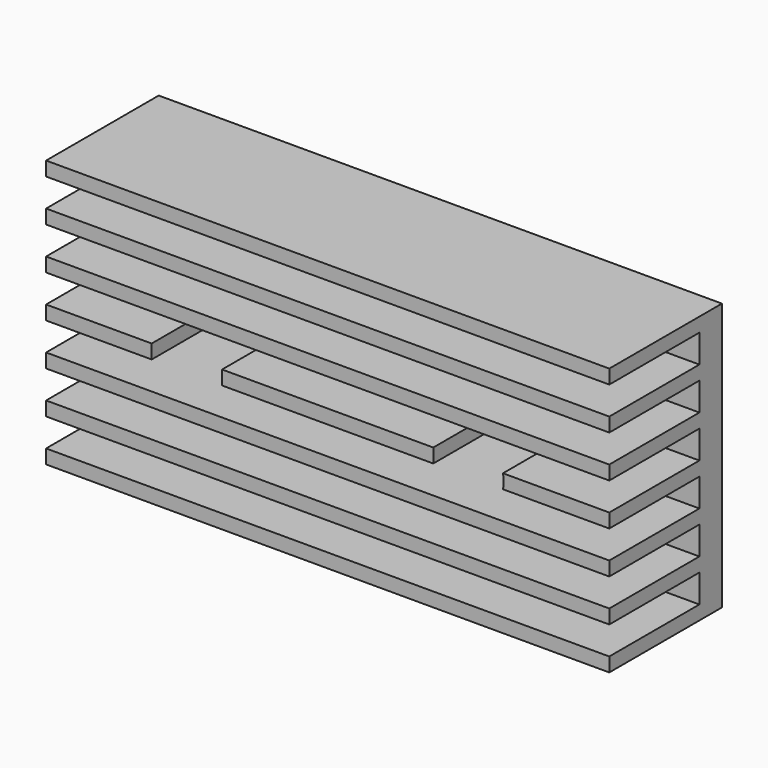
from build123d import *

# Parameters (mm, degrees)
F0_W     = 40
F0_H     = 19
F1_DEPTH = 10
F2_W     = 40
F2_H     = 2
F4_DEPTH = 8
F5_R     = 0.9
F5_W     = 4.6
F5_H     = 6.1
F7_DEPTH = 5
F8_DEPTH = 8.001
F9_DEPTH = 5.001


# Not quite as in the source:
# - a feature names something its author has since deleted; it is built from what else it names


with BuildPart() as f1:
    # F0 (on Front) → F1 (new body)
    with BuildSketch(Plane.XZ):
        Rectangle(F0_W, F0_H)
    extrude(amount=F1_DEPTH)

    # F2 (on face) → F4 (cut, through all)
    with BuildSketch(Plane.XZ.offset(10)):
        with Locations((0, 7.5)):
            Rectangle(F2_W, F2_H)
        with Locations((0, 4.5)):
            Rectangle(F2_W, F2_H)
        with Locations((0, 1.5)):
            Rectangle(F2_W, F2_H)
        with Locations((0, -1.5)):
            Rectangle(F2_W, F2_H)
        with Locations((0, -4.5)):
            Rectangle(F2_W, F2_H)
        with Locations((0, -7.5)):
            Rectangle(F2_W, F2_H)
    extrude(amount=-F4_DEPTH, mode=Mode.SUBTRACT)

    # F5 (on offset) → F7 (join, through all)
    with BuildSketch(Plane.XZ.offset(2)):
        with BuildLine():
            ThreePointArc((10, 2.5), (8.232233047, 1.767766953), (7.5, 0))
            ThreePointArc((7.5, 0), (8.232233047, -1.767766953), (10, -2.5))
            ThreePointArc((10, -2.5), (11.767766953, -1.767766953), (12.5, 0))
            ThreePointArc((12.5, 0), (11.767766953, 1.767766953), (10, 2.5))
        make_face()
        with Locations((10, 0)):
            Circle(F5_R, mode=Mode.SUBTRACT)
        with BuildLine():
            ThreePointArc((-10, -2.5), (-8.232233047, -1.767766953), (-7.5, 0))
            ThreePointArc((-7.5, 0), (-8.232233047, 1.767766953), (-10, 2.5))
            ThreePointArc((-10, 2.5), (-11.767766953, 1.767766953), (-12.5, 0))
            ThreePointArc((-12.5, 0), (-11.767766953, -1.767766953), (-10, -2.5))
        make_face()
        with Locations((-10, 0)):
            Circle(F5_R, mode=Mode.SUBTRACT)
        with Locations((0, -1.25)):
            Rectangle(F5_W, F5_H)
    extrude(amount=-F7_DEPTH)

    # F5 (on offset) → F8 (cut, through all)
    with BuildSketch(Plane.XZ.offset(2)):
        with BuildLine():
            ThreePointArc((-10, 2.5), (-8.232233047, 1.767766953), (-7.5, 0))
            Line((-7.5, 0), (-7.5, 2.5))
            Line((-7.5, 2.5), (-10, 2.5))
        make_face()
        with BuildLine():
            ThreePointArc((-12.5, 0), (-11.767766953, 1.767766953), (-10, 2.5))
            Line((-10, 2.5), (-12.5, 2.5))
            Line((-12.5, 2.5), (-12.5, 0))
        make_face()
        with BuildLine():
            Line((-12.5, -2.5), (-10, -2.5))
            ThreePointArc((-10, -2.5), (-11.767766953, -1.767766953), (-12.5, 0))
            Line((-12.5, 0), (-12.5, -2.5))
        make_face()
        with BuildLine():
            Line((-7.5, -2.5), (-7.5, 0))
            ThreePointArc((-7.5, 0), (-8.232233047, -1.767766953), (-10, -2.5))
            Line((-10, -2.5), (-7.5, -2.5))
        make_face()
        with BuildLine():
            ThreePointArc((-10, -2.5), (-8.232233047, -1.767766953), (-7.5, 0))
            ThreePointArc((-7.5, 0), (-8.232233047, 1.767766953), (-10, 2.5))
            ThreePointArc((-10, 2.5), (-11.767766953, 1.767766953), (-12.5, 0))
            ThreePointArc((-12.5, 0), (-11.767766953, -1.767766953), (-10, -2.5))
        make_face()
        with Locations((-10, 0)):
            Circle(F5_R, mode=Mode.SUBTRACT)
        with Locations((-10, 0)):
            Circle(F5_R)
        with BuildLine():
            Line((10, 2.5), (7.5, 2.5))
            Line((7.5, 2.5), (7.5, 0))
            ThreePointArc((7.5, 0), (8.232233047, 1.767766953), (10, 2.5))
        make_face()
        with BuildLine():
            ThreePointArc((10, -2.5), (8.232233047, -1.767766953), (7.5, 0))
            Line((7.5, 0), (7.5, -2.5))
            Line((7.5, -2.5), (10, -2.5))
        make_face()
        with BuildLine():
            ThreePointArc((10, 2.5), (8.232233047, 1.767766953), (7.5, 0))
            ThreePointArc((7.5, 0), (8.232233047, -1.767766953), (10, -2.5))
            ThreePointArc((10, -2.5), (11.767766953, -1.767766953), (12.5, 0))
            ThreePointArc((12.5, 0), (11.767766953, 1.767766953), (10, 2.5))
        make_face()
        with Locations((10, 0)):
            Circle(F5_R, mode=Mode.SUBTRACT)
        with Locations((10, 0)):
            Circle(F5_R)
    extrude(amount=F8_DEPTH, mode=Mode.SUBTRACT)

    # F5 (on offset) → F9 (cut, through all)
    with BuildSketch(Plane.XZ.offset(2)):
        with Locations((10, 0)):
            Circle(F5_R)
        with Locations((-10, 0)):
            Circle(F5_R)
    extrude(amount=-F9_DEPTH, mode=Mode.SUBTRACT)


solid = f1.part
